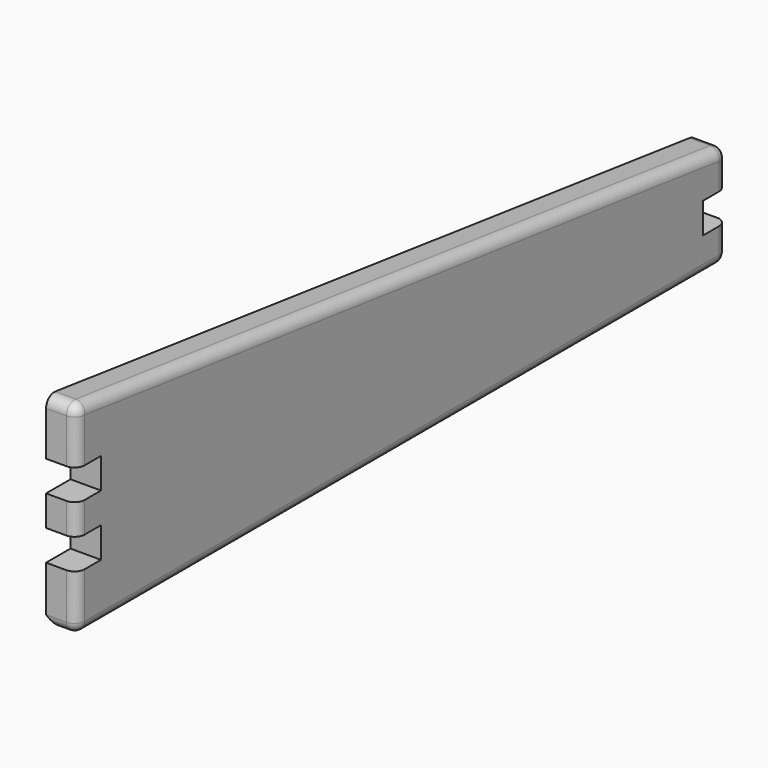
from build123d import *

# Parameters (mm, degrees)
F1_DEPTH     = 15
F2_R         = 5
F3_T1_DEPTH  = 418.0350652296
F4_T1_DEPTH  = 390
F4_T3_DEPTH  = 22.5
F4_T5_DEPTH  = 21.0347777317
F4_T7_DEPTH  = 24.1597777317
F4_T12_DEPTH = 5
F4_T18_DEPTH = 5
F4_T22_ANGLE = 90
F4_T24_ANGLE = 90
F5_T1_DEPTH  = 415.7168298797


# Not quite as in the source:
# - a fillet or chamfer that OpenCascade refuses, or shapes differently, is made with other operations: its cross-section is extruded or revolved along the edge and cut away or added


with BuildPart() as f1:
    # F0 (on Right) → F1 (new body)
    with BuildSketch(Plane.YZ):
        Polygon((-193.8978725672, -35.3695585671), (206.1021274328, -35.3695585671), (206.1021274328, -17.8695585671), (191.1021274328, -17.8695585671), (191.1021274328, -2.8695585671), (206.1021274328, -2.8695585671), (206.1021274328, 14.6304414329), (-193.8978725672, 64.6304414329), (-193.8978725672, 37.1304414329), (-178.8978725672, 37.1304414329), (-178.8978725672, 22.1304414329), (-193.8978725672, 22.1304414329), (-193.8978725672, 7.1304414329), (-178.8978725672, 7.1304414329), (-178.8978725672, -7.8695585671), (-193.8978725672, -7.8695585671), align=None)
    extrude(amount=F1_DEPTH)

    # F2
    f2_edges = [f1.edges().sort_by_distance(p)[0] for p in [
        (15, 206.102127, 5.880441),
        (15, 206.102127, -26.619559),
        (15, -193.897873, -21.619559),
        (15, -193.897873, 14.630441),
        (15, -193.897873, 50.880441),
    ]]
    fillet(f2_edges, radius=F2_R)

    # F3: fillet of radius 5 on 1 edges, made by hand

    # F3_s2 → F3_t1 (cut)
    with BuildSketch(Plane(origin=(0, 208.5341292164, -26.0667661521), x_dir=(1, 0, 0), z_dir=(0, -0.9922778767, 0.1240347346))):
        with BuildLine():
            ThreePointArc((15, 35.0812860348), (13.5355339059, 38.6168199408), (10, 40.0812860348))
            Line((10, 40.0812860348), (15, 40.0812860348))
            Line((15, 40.0812860348), (15, 35.0812860348))
        make_face()
    extrude(amount=F3_T1_DEPTH, mode=Mode.SUBTRACT)

    # F4: fillet of radius 5 on 7 edges, made by hand

    # F4_s2 → F4_t1 (cut)
    with BuildSketch(Plane.XZ.offset(-201.1021274328)):
        with BuildLine():
            ThreePointArc((15, -30.3695585671), (13.5355339059, -33.905092473), (10, -35.3695585671))
            Line((10, -35.3695585671), (15, -35.3695585671))
            Line((15, -35.3695585671), (15, -30.3695585671))
        make_face()
    extrude(amount=F4_T1_DEPTH, mode=Mode.SUBTRACT)

    # F4_s4 → F4_t3 (cut)
    with BuildSketch(Plane.YZ.offset(-12.5)):
        with BuildLine():
            ThreePointArc((-193.8978725672, -30.3695585671), (-192.4334064731, -33.905092473), (-188.8978725672, -35.3695585671))
            Line((-188.8978725672, -35.3695585671), (-193.8978725672, -35.3695585671))
            Line((-193.8978725672, -35.3695585671), (-193.8978725672, -30.3695585671))
        make_face()
        with BuildLine():
            ThreePointArc((201.1021274328, -35.3695585671), (204.6376613388, -33.905092473), (206.1021274328, -30.3695585671))
            Line((206.1021274328, -30.3695585671), (206.1021274328, -35.3695585671))
            Line((206.1021274328, -35.3695585671), (201.1021274328, -35.3695585671))
        make_face()
    extrude(amount=F4_T3_DEPTH, mode=Mode.SUBTRACT)

    # F4_s6 → F4_t5 (cut)
    with BuildSketch(Plane.YZ.offset(-11.0347777317)):
        with BuildLine():
            ThreePointArc((206.1021274328, 10.2165303402), (204.8505183119, 13.5255431564), (201.7223011058, 15.1779197238))
            Line((201.7223011058, 15.1779197238), (206.1021274328, 14.6304414329))
            Line((206.1021274328, 14.6304414329), (206.1021274328, 10.2165303402))
        make_face()
    extrude(amount=F4_T5_DEPTH, mode=Mode.SUBTRACT)

    # F4_s8 → F4_t7 (cut)
    with BuildSketch(Plane.YZ.offset(-14.1597777317)):
        with BuildLine():
            ThreePointArc((-188.2776988942, 63.9279197238), (-192.2068853834, 62.7149212193), (-193.8978725672, 58.9665303402))
            Line((-193.8978725672, 58.9665303402), (-193.8978725672, 64.6304414329))
            Line((-193.8978725672, 64.6304414329), (-188.2776988942, 63.9279197238))
        make_face()
    extrude(amount=F4_T7_DEPTH, mode=Mode.SUBTRACT)


with BuildPart() as f4_tool10:
    # F4_s11 → F4_t12 (new body)
    with BuildSketch(Plane.YZ.offset(10)):
        Polygon((-188.8978725672, 58.9665303402), (-188.2776988942, 63.9279197238), (-193.8978725672, 64.6304414329), (-193.8978725672, 58.9665303402), align=None)
    extrude(amount=F4_T12_DEPTH)

    # F4_s13 → F4_t14 (revolve, cut)
    with BuildSketch(Plane(origin=(10, -188.8978725672, 58.9665303402), x_dir=(0, 0.6618025632, -0.7496781758), z_dir=(0, -0.7496781758, -0.6618025632))):
        with BuildLine():
            ThreePointArc((0, -5), (5, 0), (0, 5))
            Line((0, 5), (0, -5))
        make_face()
    revolve(axis=Axis((10, -188.8978725672, 58.9665303402), (1, 0, 0)), mode=Mode.SUBTRACT)


with BuildPart() as f1_1:
    add(f1.part)

    # F4_t9: cut F4_tool10
    add(f4_tool10.part, mode=Mode.SUBTRACT)


with BuildPart() as f4_tool16:
    # F4_s17 → F4_t18 (new body)
    with BuildSketch(Plane.YZ.offset(10)):
        Polygon((201.1021274328, 10.2165303402), (206.1021274328, 10.2165303402), (206.1021274328, 14.6304414329), (201.7223011058, 15.1779197238), align=None)
    extrude(amount=F4_T18_DEPTH)

    # F4_s19 → F4_t20 (revolve, cut)
    with BuildSketch(Plane(origin=(10, 201.1021274328, 10.2165303402), x_dir=(0, -0.7496781758, -0.6618025632), z_dir=(0, -0.6618025632, 0.7496781758))):
        with BuildLine():
            ThreePointArc((0, -5), (5, 0), (0, 5))
            Line((0, 5), (0, -5))
        make_face()
    revolve(axis=Axis((10, 201.1021274328, 10.2165303402), (1, 0, 0)), mode=Mode.SUBTRACT)


with BuildPart() as f1_2:
    add(f1_1.part)

    # F4_t15: cut F4_tool16
    add(f4_tool16.part, mode=Mode.SUBTRACT)

    # F4_s21 → F4_t22 (revolve, cut)
    with BuildSketch(Plane.YZ.offset(10)):
        with BuildLine():
            ThreePointArc((-188.8978725672, -35.3695585671), (-192.4334064731, -33.905092473), (-193.8978725672, -30.3695585671))
            Line((-193.8978725672, -30.3695585671), (-193.8978725672, -35.3695585671))
            Line((-193.8978725672, -35.3695585671), (-188.8978725672, -35.3695585671))
        make_face()
    revolve(axis=Axis((10, -188.8978725672, -35.3695585671), (0, 0, 1)), revolution_arc=F4_T22_ANGLE, mode=Mode.SUBTRACT)

    # F4_s23 → F4_t24 (revolve, cut)
    with BuildSketch(Plane.YZ.offset(10)):
        with BuildLine():
            ThreePointArc((201.1021274328, -35.3695585671), (204.6376613388, -33.905092473), (206.1021274328, -30.3695585671))
            Line((206.1021274328, -30.3695585671), (206.1021274328, -35.3695585671))
            Line((206.1021274328, -35.3695585671), (201.1021274328, -35.3695585671))
        make_face()
    revolve(axis=Axis((10, 201.1021274328, -35.3695585671), (0, 0, -1)), revolution_arc=F4_T24_ANGLE, mode=Mode.SUBTRACT)

    # F5: chamfer of 5 on 1 edges, made by hand

    # F5_s2 → F5_t1 (cut)
    with BuildSketch(Plane.XZ.offset(-213.9605423726)):
        Polygon((0, -30.3695585671), (5, -35.3695585671), (0, -35.3695585671), align=None)
    extrude(amount=F5_T1_DEPTH, mode=Mode.SUBTRACT)


solid = f1_2.part
